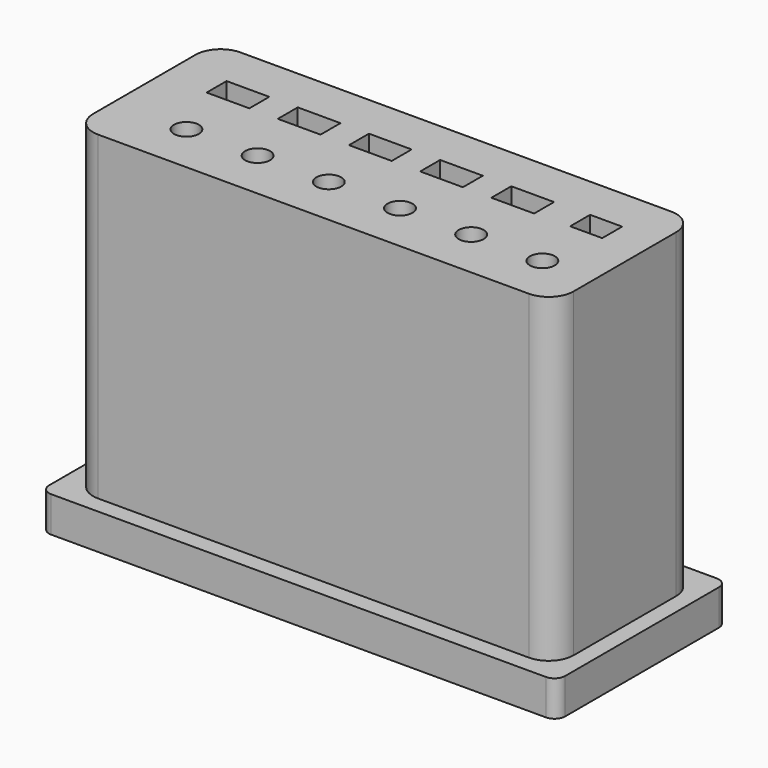
from build123d import *

# Parameters (mm, degrees)
F0_W     = 135
F0_H     = 100
F1_DEPTH = 50
F2_W     = 12
F2_H     = 7
F2_W_2   = 9
F3_DEPTH = 75
F5_D     = 7
F5_DEPTH = 52
F5_TIP   = 2.1030121666
F6_W     = 145
F6_H     = 60
F7_DEPTH = 10
F8_R     = 7
F9_R     = 3


# Not quite as in the source:
# - a feature names something its author has since deleted; it is built from what else it names


with BuildPart() as f1:
    # F0 (on Front) → F1 (new body)
    with BuildSketch(Plane.XZ):
        with Locations((67.5, 50)):
            Rectangle(F0_W, F0_H)
    extrude(amount=F1_DEPTH)

    # F2 (on face) → F3 (cut)
    with BuildSketch(Plane.XY.offset(100)):
        with Locations((19.1170862466, -16.0328453556)):
            Rectangle(F2_W, F2_H)
        with Locations((39.1170862466, -16.0328453556)):
            Rectangle(F2_W, F2_H)
        with Locations((59.1170862466, -16.0328453556)):
            Rectangle(F2_W, F2_H)
        with Locations((79.1170862466, -16.0328453556)):
            Rectangle(F2_W, F2_H)
        with Locations((99.1170862466, -16.0328453556)):
            Rectangle(F2_W, F2_H)
        with Locations((119.5874011219, -15.8250607699)):
            Rectangle(F2_W_2, F2_H)
    extrude(amount=-F3_DEPTH, mode=Mode.SUBTRACT)

    # F5
    with Locations(Plane.XY.offset(100)):
        with Locations((20.5715699643, -35.9477512538), (40.5715699643, -35.9477512538), (60.5715699643, -35.9477512538), (80.5715699643, -35.9477512538), (100.5715699643, -35.9477512538), (120.5715699643, -35.9477512538)):
            Hole(F5_D / 2, depth=F5_DEPTH)
            with Locations((0, 0, -(F5_DEPTH + F5_TIP / 2))):  # 118° drill point
                Cone(0, F5_D / 2, F5_TIP, mode=Mode.SUBTRACT)

    # F6 (on Top) → F7 (join)
    with BuildSketch(Plane.XY):
        with Locations((67.1998835728, -24.8457092833)):
            Rectangle(F6_W, F6_H)
    extrude(amount=F7_DEPTH)

    # F8
    f8_edges = [f1.edges().sort_by_distance(p)[0] for p in [
        (0, -50, 55),
        (135, -50, 55),
        (135, 0, 55),
        (0, 0, 55),
    ]]
    fillet(f8_edges, radius=F8_R)

    # F9
    f9_edges = [f1.edges().sort_by_distance(p)[0] for p in [
        (-5.300116, 5.154291, 5),
        (-5.300116, -54.845709, 5),
        (139.699884, -54.845709, 5),
        (139.699884, 5.154291, 5),
    ]]
    fillet(f9_edges, radius=F9_R)


solid = f1.part
